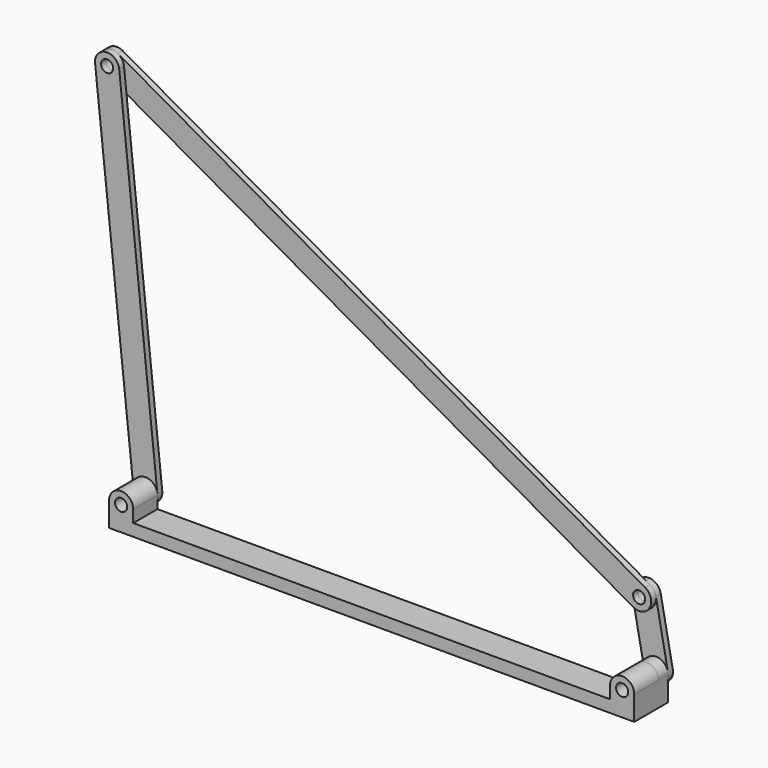
from build123d import *

# Parameters (mm, degrees)
F0_R     = 0.254
F1_DEPTH = 1.27
F2_R     = 0.254
F3_DEPTH = 0.254
F4_R     = 0.254
F5_DEPTH = 0.254
F6_R     = 0.254
F7_DEPTH = 0.254
F8_R     = 0.254
F9_DEPTH = 0.508


with BuildPart() as f1:
    # F0 (on Front) → F1 (new body)
    with BuildSketch(Plane.XZ):
        with BuildLine():
            Line((0, 1.016), (0, 0.508))
            Line((0, 0.508), (1.016, 0.508))
            Line((1.016, 0.508), (1.016, 1.016))
            ThreePointArc((1.016, 1.016), (0.508, 1.524), (0, 1.016))
        make_face()
        with Locations((0.508, 1.016)):
            Circle(F0_R, mode=Mode.SUBTRACT)
        Polygon((0, 0.508), (0, 0), (22.0218, 0), (22.0218, 0.508), (21.0058, 0.508), (1.016, 0.508), align=None)
        with BuildLine():
            Line((21.0058, 0.508), (22.0218, 0.508))
            Line((22.0218, 0.508), (22.0218, 1.016))
            ThreePointArc((22.0218, 1.016), (21.5138, 1.524), (21.0058, 1.016))
            Line((21.0058, 1.016), (21.0058, 0.508))
        make_face()
        with Locations((21.5138, 1.016)):
            Circle(F0_R, mode=Mode.SUBTRACT)
    extrude(amount=F1_DEPTH)

    # F8 (on face) → F9 (join)
    with BuildSketch(Plane(origin=(0, 0, 0), x_dir=(-1, 0, 0), z_dir=(0, 1, 0))):
        with BuildLine():
            ThreePointArc((-22.0126938926, 1.1117542892), (-22.0195183492, 1.064093152), (-22.0218, 1.016))
            Line((-22.0218, 1.016), (-22.0218, 0.508))
            Line((-22.0218, 0.508), (-22.0218, 0))
            Line((-22.0218, 0), (-21.0058, 0))
            Line((-21.0058, 0), (-21.0058, 0.508))
            Line((-21.0058, 0.508), (-21.0058, 1.016))
            ThreePointArc((-21.0058, 1.016), (-21.465706848, 1.5217183492), (-22.0126938926, 1.1117542892))
        make_face()
        with Locations((-21.5138, 1.016)):
            Circle(F8_R, mode=Mode.SUBTRACT)
    extrude(amount=F9_DEPTH)


with BuildPart() as f3:
    # F2 (on face) → F3 (new body)
    with BuildSketch(Plane(origin=(0, 0, 0), x_dir=(-1, 0, 0), z_dir=(0, 1, 0))):
        with BuildLine():
            ThreePointArc((-1.0131799286, 1.0694531545), (-0.5347637466, 0.5087055077), (0, 1.016))
            ThreePointArc((0, 1.016), (-0.4812362534, 1.5232944923), (-1.0131799286, 1.0694531545))
        make_face()
        with Locations((-0.508, 1.016)):
            Circle(F2_R, mode=Mode.SUBTRACT)
        with BuildLine():
            ThreePointArc((-1.0131799286, 1.0694531545), (-0.4812362534, 1.5232944923), (0, 1.016))
            Line((0, 1.016), (1.6007646277, 16.1178508951))
            ThreePointArc((1.6007646277, 16.1178508951), (1.0420945746, 15.6662228951), (0.5904147052, 16.224851013))
            Line((0.5904147052, 16.224851013), (-1.0131799286, 1.0694531545))
        make_face()
        with BuildLine():
            ThreePointArc((0.5904147052, 16.224851013), (1.0420945746, 15.6662228951), (1.6007646277, 16.1178508951))
            ThreePointArc((1.6007646277, 16.1178508951), (1.6028866389, 16.1445870108), (1.6035946338, 16.1713978585))
            ThreePointArc((1.6035946338, 16.1713978585), (1.1223583804, 16.6786923508), (0.5904147052, 16.224851013))
        make_face()
        with Locations((1.0955946338, 16.1713978585)):
            Circle(F2_R, mode=Mode.SUBTRACT)
    extrude(amount=F3_DEPTH)


with BuildPart() as f5:
    # F4 (on face) → F5 (new body)
    with BuildSketch(Plane(origin=(0, 0.254, 0), x_dir=(-1, 0, 0), z_dir=(0, 1, 0))):
        with BuildLine():
            ThreePointArc((1.3459001233, 15.7293445112), (1.5344677297, 15.9155572721), (1.6035946338, 16.1713978585))
            ThreePointArc((1.6035946338, 16.1713978585), (1.3514352202, 16.6102709545), (0.8452891443, 16.6134512059))
            ThreePointArc((0.8452891443, 16.6134512059), (0.6535412864, 15.921092369), (1.3459001233, 15.7293445112))
        make_face()
        with Locations((1.0955946338, 16.1713978585)):
            Circle(F4_R, mode=Mode.SUBTRACT)
        with BuildLine():
            ThreePointArc((1.3459001233, 15.7293445112), (0.6535412864, 15.921092369), (0.8452891443, 16.6134512059))
            Line((0.8452891443, 16.6134512059), (-21.2573782243, 4.0981767306))
            ThreePointArc((-21.2573782243, 4.0981767306), (-20.7512321484, 4.0949964791), (-20.4990727348, 3.6561233832))
            ThreePointArc((-20.4990727348, 3.6561233832), (-20.5681996389, 3.4002827968), (-20.7567672453, 3.2140700358))
            Line((-20.7567672453, 3.2140700358), (1.3459001233, 15.7293445112))
        make_face()
        with BuildLine():
            ThreePointArc((-20.4990727348, 3.6561233832), (-20.7512321484, 4.0949964791), (-21.2573782243, 4.0981767306))
            ThreePointArc((-21.2573782243, 4.0981767306), (-21.4491260822, 3.4058178937), (-20.7567672453, 3.2140700358))
            ThreePointArc((-20.7567672453, 3.2140700358), (-20.5681996389, 3.4002827968), (-20.4990727348, 3.6561233832))
        make_face()
        with Locations((-21.0070727348, 3.6561233832)):
            Circle(F4_R, mode=Mode.SUBTRACT)
    extrude(amount=F5_DEPTH)


with BuildPart() as f7:
    # F6 (on face) → F7 (new body)
    with BuildSketch(Plane(origin=(0, 0.508, 0), x_dir=(-1, 0, 0), z_dir=(0, 1, 0))):
        with BuildLine():
            ThreePointArc((-20.5081788422, 3.5603690941), (-20.5013543856, 3.6080302312), (-20.4990727348, 3.6561233832))
            ThreePointArc((-20.4990727348, 3.6561233832), (-20.9589795828, 4.1618417324), (-21.5059666274, 3.7518776724))
            ThreePointArc((-21.5059666274, 3.7518776724), (-21.102827024, 3.1572294906), (-20.5081788422, 3.5603690941))
        make_face()
        with Locations((-21.0070727348, 3.6561233832)):
            Circle(F6_R, mode=Mode.SUBTRACT)
        with BuildLine():
            ThreePointArc((-20.5081788422, 3.5603690941), (-21.102827024, 3.1572294906), (-21.5059666274, 3.7518776724))
            Line((-21.5059666274, 3.7518776724), (-22.0126938926, 1.1117542892))
            ThreePointArc((-22.0126938926, 1.1117542892), (-21.465706848, 1.5217183492), (-21.0058, 1.016))
            ThreePointArc((-21.0058, 1.016), (-21.0080816508, 0.967906848), (-21.0149061074, 0.9202457108))
            Line((-21.0149061074, 0.9202457108), (-20.5081788422, 3.5603690941))
        make_face()
        with BuildLine():
            ThreePointArc((-21.0058, 1.016), (-21.465706848, 1.5217183492), (-22.0126938926, 1.1117542892))
            ThreePointArc((-22.0126938926, 1.1117542892), (-21.6095542892, 0.5171061074), (-21.0149061074, 0.9202457108))
            ThreePointArc((-21.0149061074, 0.9202457108), (-21.0080816508, 0.967906848), (-21.0058, 1.016))
        make_face()
        with Locations((-21.5138, 1.016)):
            Circle(F6_R, mode=Mode.SUBTRACT)
    extrude(amount=F7_DEPTH)


solid = Compound([f1.part, f3.part, f5.part, f7.part])
